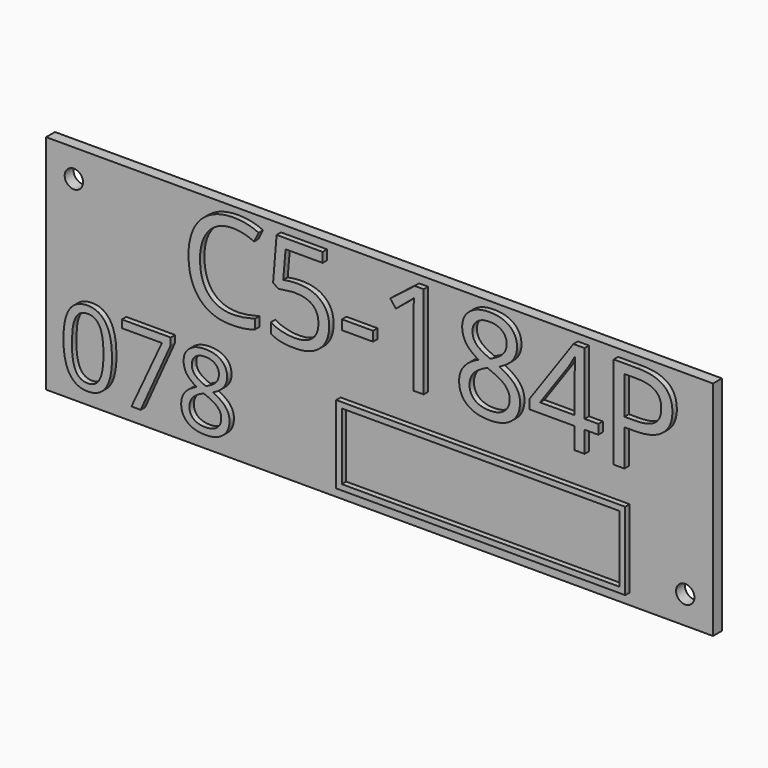
from build123d import *

# Parameters (mm, degrees)
F0_W         = 120
F0_H         = 40
F1_DEPTH     = 2
F3_D         = 3.3
F4_TEXT_SIZE = 23.3453572731
F5_DEPTH     = 1
F6_TEXT_SIZE = 18.5155049272
F7_DEPTH     = 1
F8_W         = 52
F8_H         = 14
F8_W_2       = 49.99999962
F8_H_2       = 11.99999962
F9_DEPTH     = 1


# Not quite as in the source:
# - Text() gives the source's letters only with a copy of the font that has no kerning and outlines rounded to 1/6400 em; it was checked with that copy


with BuildPart() as f1:
    # F0 (on Front) → F1 (new body)
    with BuildSketch(Plane.XZ):
        Rectangle(F0_W, F0_H)
    extrude(amount=F1_DEPTH)

    # F3 (through all)
    with Locations(Plane.XZ.offset(2)):
        with Locations((-55, 15), (55, -15)):
            Hole(F3_D / 2)

    # F4 (on face) → F5 (join)
    with BuildSketch(Plane.XZ.offset(2)):
        with Locations((-35, 2)):
            Text('C5-184P', F4_TEXT_SIZE, font='Open Sans', text_align=(TextAlign.LEFT, TextAlign.BOTTOM))
    extrude(amount=F5_DEPTH)

    # F6 (on face) → F7 (join)
    with BuildSketch(Plane.XZ.offset(2)):
        with Locations((-57, -17)):
            Text('078', F6_TEXT_SIZE, font='Open Sans', text_align=(TextAlign.LEFT, TextAlign.BOTTOM))
    extrude(amount=F7_DEPTH)

    # F8 (on face) → F9 (join)
    with BuildSketch(Plane.XZ.offset(2)):
        with Locations((19, -11)):
            Rectangle(F8_W, F8_H)
        with Locations((19, -11)):
            Rectangle(F8_W_2, F8_H_2, mode=Mode.SUBTRACT)
    extrude(amount=F9_DEPTH)


solid = f1.part
